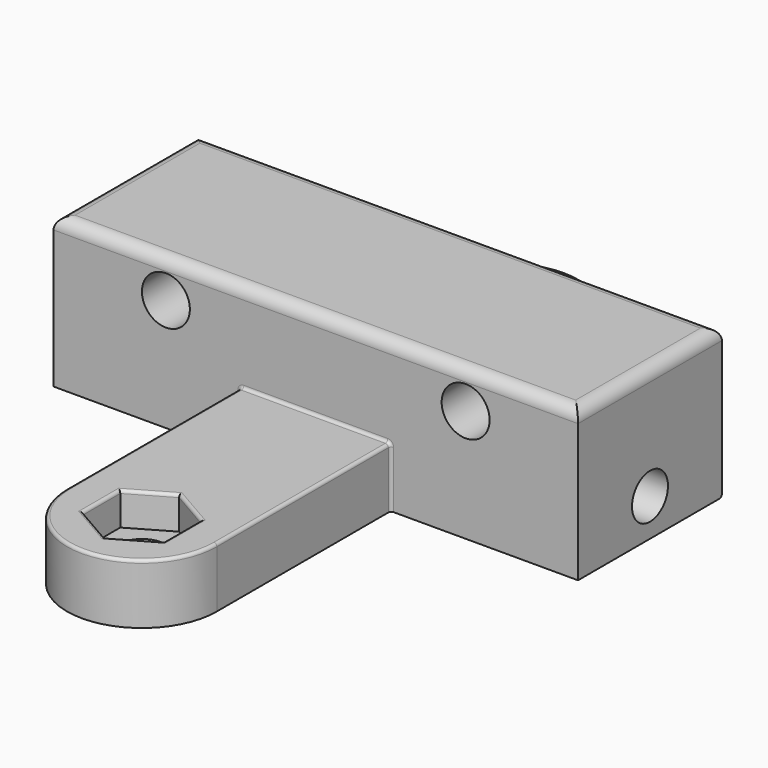
from build123d import *

# Parameters (mm, degrees)
F0_R      = 1.6
F1_DEPTH  = 4
F2_W      = 35
F2_H      = 12
F3_DEPTH  = 6
F4_R      = 1.6
F5_DEPTH  = 20.751
F6_R      = 0.8
F7_R      = 1.5
F8_DEPTH  = 35.001
F10_DEPTH = 2.2
F11_R     = 0.2


with BuildPart() as f1:
    # F0 (on Top) → F1 (new body)
    with BuildSketch(Plane.XY):
        with BuildLine():
            ThreePointArc((5, 30.25), (0, 35.25), (-5, 30.25))
            Line((-5, 30.25), (-5, 26.5))
            Line((-5, 26.5), (-17.5, 26.5))
            Line((-17.5, 26.5), (-17.5, 14.5))
            Line((-17.5, 14.5), (-5, 14.5))
            Line((-5, 14.5), (-5, 0))
            ThreePointArc((-5, 0), (0, -5), (5, 0))
            Line((5, 0), (5, 14.5))
            Line((5, 14.5), (17.5, 14.5))
            Line((17.5, 14.5), (17.5, 26.5))
            Line((17.5, 26.5), (5, 26.5))
            Line((5, 26.5), (5, 30.25))
        make_face()
        Circle(F0_R, mode=Mode.SUBTRACT)
        with Locations((0, 30.25)):
            Circle(F0_R, mode=Mode.SUBTRACT)
    extrude(amount=F1_DEPTH)

    # F2 (on face) → F3 (join)
    with BuildSketch(Plane.XY.offset(4)):
        with Locations((0, 20.5)):
            Rectangle(F2_W, F2_H)
    extrude(amount=F3_DEPTH)

    # F4 (on face) → F5 (cut, through all)
    with BuildSketch(Plane.XZ.offset(-14.5)):
        with Locations((-10, 7.5)):
            Circle(F4_R)
        with Locations((10, 7.5)):
            Circle(F4_R)
    extrude(amount=-F5_DEPTH, mode=Mode.SUBTRACT)

    # F6
    f6_edges = [f1.edges().sort_by_distance(p)[0] for p in [
        (0, 26.5, 10),
        (-17.5, 20.5, 10),
        (0, 14.5, 10),
        (17.5, 20.5, 10),
    ]]
    fillet(f6_edges, radius=F6_R)

    # F7 (on face) → F8 (cut, through all)
    with BuildSketch(Plane.YZ.offset(17.5)):
        with Locations((20.5, 2.5)):
            Circle(F7_R)
    extrude(amount=-F8_DEPTH, mode=Mode.SUBTRACT)

    # F9 (on face) → F10 (cut)
    with BuildSketch(Plane.XY.offset(4)):
        Polygon((-2.6846787517, 28.7), (0, 27.15), (2.6846787517, 28.7), (2.6846787517, 31.8), (0, 33.35), (-2.6846787517, 31.8), align=None)
        Polygon((2.6846787517, 1.55), (0, 3.1), (-2.6846787517, 1.55), (-2.6846787517, -1.55), (0, -3.1), (2.6846787517, -1.55), align=None)
    extrude(amount=-F10_DEPTH, mode=Mode.SUBTRACT)

    # F11
    f11_edges = [f1.edges().sort_by_distance(p)[0] for p in [
        (5, 7.25, 4),
        (0, -5, 4),
        (0, 14.5, 4),
        (-5, 7.25, 4),
        (2.684679, 0, 4),
        (1.342339, 2.325, 4),
        (-1.342339, 2.325, 4),
        (-2.684679, 0, 4),
        (-1.342339, -2.325, 4),
        (1.342339, -2.325, 4),
        (5, 28.375, 4),
        (0, 26.5, 4),
        (0, 35.25, 4),
        (-5, 28.375, 4),
        (-1.342339, 27.925, 4),
        (1.342339, 27.925, 4),
        (2.684679, 30.25, 4),
        (1.342339, 32.575, 4),
        (-1.342339, 32.575, 4),
        (-2.684679, 30.25, 4),
        (-5, 30.25, 2),
        (-5, 26.5, 2),
        (-5, 28.375, 0),
        (11.25, 26.5, 0),
        (5, 26.5, 2),
        (-11.25, 26.5, 0),
        (0, 35.25, 0),
        (5, 28.375, 0),
        (-5, 14.5, 2),
        (5, 14.5, 2),
    ]]
    fillet(f11_edges, radius=F11_R)


solid = f1.part
